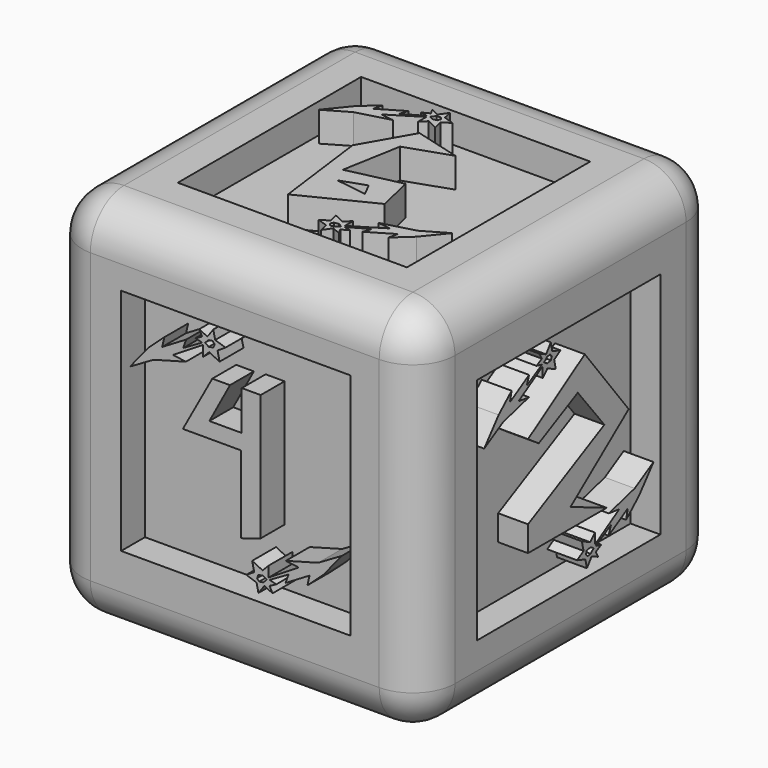
from build123d import *

# Parameters (mm, degrees)
F0_W      = 12.5
F0_H      = 12.5
F1_DEPTH  = 12.5
F2_R      = 1.4103835631
F3_W      = 7.6792328737
F3_H      = 7.6792328737
F4_DEPTH  = 1
F5_W      = 7.6792328737
F5_H      = 7.6792328737
F6_DEPTH  = 1
F7_W      = 7.6792328737
F7_H      = 7.6792328737
F8_DEPTH  = 1
F9_W      = 7.6792328737
F9_H      = 7.6792328737
F10_DEPTH = 1
F12_W     = 7.6792328737
F12_H     = 7.6792328737
F13_DEPTH = 1
F14_W     = 7.6792328737
F14_H     = 7.6792328737
F15_DEPTH = 1


# Not quite as in the source:
# - a feature names something its author has since deleted; it is built from what else it names


with BuildPart() as f1:
    # F0 (on Front) → F1 (new body)
    with BuildSketch(Plane.XZ):
        with Locations((0.0040858053, -0.2807128243)):
            Rectangle(F0_W, F0_H)
    extrude(amount=F1_DEPTH)

    # F2
    f2_edges = [f1.edges().sort_by_distance(p)[0] for p in [
        (-6.245914, -6.25, 5.969287),
        (6.254086, -6.25, 5.969287),
        (0.004086, 0, 5.969287),
        (0.004086, -12.5, 5.969287),
        (-6.245914, -6.25, -6.530713),
        (6.254086, -6.25, -6.530713),
        (0.004086, 0, -6.530713),
        (0.004086, -12.5, -6.530713),
        (6.254086, -12.5, -0.280713),
        (-6.245914, -12.5, -0.280713),
        (6.254086, 0, -0.280713),
        (-6.245914, 0, -0.280713),
    ]]
    fillet(f2_edges, radius=F2_R)

    # F3 (on face) → F4 (cut)
    with BuildSketch(Plane.XY.offset(5.9692871757)):
        with Locations((0.0040858053, -6.25)):
            Rectangle(F3_W, F3_H)
        Polygon((-0.652328541, -3.9411829785), (0.8822005475, -4.3596909381), (-0.5726128584, -4.8579145223), (-0.9213888927, -6.8151349505), (0.8622713503, -6.4123724587), (1.141276909, -7.647966966), (-1.1704812059, -8.8038453832), (-1.5889889328, -5.5753565393), align=None, mode=Mode.SUBTRACT)
        Polygon((3.5567511804, -7.8321555629), (2.9507998843, -8.5790259764), (2.4082618766, -9.0722423047), (2.4787215516, -8.7622206192), (1.6754835378, -9.2413448729), (1.7741267802, -8.959507104), (1.1399915675, -9.325896157), (1.3654618524, -9.3822639901), (1.1399915675, -9.5020448789), (1.2393376978, -9.6890496718), (0.9638429037, -9.5584124792), (0.766556419, -9.83320456), (0.7031428395, -9.5443206374), (0.3578914911, -9.4315854367), (0.6256374181, -9.2624826357), (0.5551779759, -8.9524611831), (0.9074754198, -9.1215639841), (1.1047618464, -8.9172313455), (1.1047618464, -9.2695287894), (2.1193781868, -8.6424394976), (1.6825294588, -8.5860718973), (2.7676052414, -8.2901422866), align=None, mode=Mode.SUBTRACT)
        Polygon((-3.5365826916, -4.553236533), (-2.9306313954, -3.8063661195), (-2.3880933877, -3.3131497912), (-2.4585530628, -3.6231714766), (-1.655315049, -3.144047223), (-1.7539582914, -3.4258849919), (-1.1198230786, -3.0594959389), (-1.3452933636, -3.0031281058), (-1.1198230786, -2.883347217), (-1.2191692089, -2.696342424), (-0.9436744149, -2.8269796167), (-0.7463879301, -2.5521875359), (-0.6829743506, -2.8410714585), (-0.3377230023, -2.9538066592), (-0.6054689293, -3.1229094602), (-0.5350094871, -3.4329309128), (-0.887306931, -3.2638281118), (-1.0845933575, -3.4681607503), (-1.0845933575, -3.1158633064), (-2.0992096979, -3.7429525983), (-1.6623609699, -3.7993201986), (-2.7474367525, -4.0952498093), align=None, mode=Mode.SUBTRACT)
        Polygon((0.7911975845, -9.4897663221), (0.9244724642, -9.4698371831), (1.0452916613, -9.3527548015), (0.918244652, -9.2730389442), (0.7637953386, -9.3004412483), (0.7214463549, -9.4112961087), align=None)
        Polygon((-0.7710290956, -2.8956257738), (-0.9043039754, -2.9155549128), (-1.0251231724, -3.0326372944), (-0.8980761631, -3.1123531517), (-0.7436268497, -3.0849508476), (-0.701277866, -2.9740959872), align=None)
        Polygon((0.3839768178, -7.5283930637), (0.1647583413, -7.0899561979), (-0.6642947193, -7.3738783735), align=None)
    extrude(amount=-F4_DEPTH, mode=Mode.SUBTRACT)

    # F5 (on face) → F6 (cut)
    with BuildSketch(Plane(origin=(0, 0, 0), x_dir=(-1, 0, 0), z_dir=(0, 1, 0))):
        with Locations((-0.1059367728, -0.2820717577)):
            Rectangle(F5_W, F5_H)
        Polygon((3.4467286024, -1.8642273206), (2.8407773062, -2.6110977341), (2.2982392985, -3.1043140624), (2.3686989736, -2.794292377), (1.5654609598, -3.2734166306), (1.6641042022, -2.9915788617), (1.0299689894, -3.3579679147), (1.2554392744, -3.4143357478), (1.0299689894, -3.5341166366), (1.1293151197, -3.7211214296), (0.8538203257, -3.5904842369), (0.6565338409, -3.8652763177), (0.5931202614, -3.5763923951), (0.2478689131, -3.4636571944), (0.5156148401, -3.2945543934), (0.4451553979, -2.9845329408), (0.7974528418, -3.1536357418), (0.9947392683, -2.9493031033), (0.9947392683, -3.3016005472), (2.0093556087, -2.6745112553), (1.5725068807, -2.618143655), (2.6575826633, -2.3222140443), align=None, mode=Mode.SUBTRACT)
        Polygon((-0.8451312315, 1.7336877688), (-0.8451312315, 2.2153509256), (2.2446786681, 0.9617710281), (0.5813771522, -0.5256042938), (1.8385423364, -1.4611691033), (-0.8458287511, -3.1528016366), (-1.0901629205, -2.8107338108), (0.9133041001, -1.3796858916), (-0.5255040818, -0.3914135535), (1.2028907008, 0.4810142225), align=None, mode=Mode.SUBTRACT)
        Polygon((-3.6466052696, 1.4146917093), (-3.0406539735, 2.1615621228), (-2.4981159657, 2.6547784511), (-2.5685756408, 2.3447567656), (-1.765337627, 2.8238810193), (-1.8639808694, 2.5420432504), (-1.2298456567, 2.9084323033), (-1.4553159416, 2.9648001365), (-1.2298456567, 3.0845810253), (-1.329191787, 3.2715858182), (-1.0536969929, 3.1409486256), (-0.8564105082, 3.4157407064), (-0.7929969287, 3.1268567838), (-0.4477455803, 3.0141215831), (-0.7154915073, 2.8450187821), (-0.6450320651, 2.5349973295), (-0.997329509, 2.7041001305), (-1.1946159356, 2.4997674919), (-1.1946159356, 2.8520649358), (-2.209232276, 2.224975644), (-1.772383548, 2.1686080437), (-2.8574593306, 1.872678433), align=None, mode=Mode.SUBTRACT)
        Polygon((-0.8810516737, 3.0723024685), (-1.0143265534, 3.0523733295), (-1.1351457505, 2.9352909479), (-1.0080987412, 2.8555750906), (-0.8536494278, 2.8829773947), (-0.8113004441, 2.9938322551), align=None)
        Polygon((0.6811750064, -3.5218380798), (0.8144498862, -3.5019089408), (0.9352690832, -3.3848265592), (0.8082220739, -3.3051107019), (0.6537727605, -3.3325130061), (0.6114237768, -3.4433678664), align=None)
    extrude(amount=-F6_DEPTH, mode=Mode.SUBTRACT)

    # F7 (on face) → F8 (cut)
    with BuildSketch(Plane(origin=(0, 0, -6.5307128243), x_dir=(1, 0, 0), z_dir=(0, 0, -1))):
        with Locations((0.0040858053, 6.25)):
            Rectangle(F7_W, F7_H)
        Polygon((3.7880760211, 4.7270533688), (3.182124725, 3.9801829554), (2.6395867172, 3.4869666271), (2.7100463923, 3.7969883125), (1.9068083785, 3.3178640589), (2.0054516209, 3.5997018277), (1.3713164082, 3.2333127748), (1.5967866931, 3.1769449416), (1.3713164082, 3.0571640529), (1.4706625385, 2.8701592599), (1.1951677444, 3.0007964525), (0.9978812597, 2.7260043718), (0.9344676802, 3.0148882944), (0.5892163318, 3.1276234951), (0.8569622588, 3.2967262961), (0.7865028166, 3.6067477487), (1.1388002605, 3.4376449477), (1.3360866871, 3.6419775862), (1.3360866871, 3.2896801423), (2.3507030274, 3.9167694341), (1.9138542995, 3.9731370345), (2.9989300821, 4.2690666452), align=None, mode=Mode.SUBTRACT)
        Polygon((-0.234052015, 8.3048082888), (-0.8038301021, 8.3048082888), (0, 9.1091999784), (0.5368242273, 9.1091999784), (0.5368242273, 3.8303739857), (-0.234052015, 3.8303739857), align=None, mode=Mode.SUBTRACT)
        Polygon((-3.7074539285, 7.7881164908), (-3.1015026324, 8.5349869042), (-2.5589646247, 9.0282032326), (-2.6294242997, 8.7181815471), (-1.8261862859, 9.1973058007), (-1.9248295283, 8.9154680319), (-1.2906943156, 9.2818570848), (-1.5161646005, 9.338224918), (-1.2906943156, 9.4580058068), (-1.3900404459, 9.6450105997), (-1.1145456518, 9.5143734071), (-0.9172591671, 9.7891654879), (-0.8538455876, 9.5002815652), (-0.5085942392, 9.3875463646), (-0.7763401662, 9.2184435636), (-0.705880724, 8.908422111), (-1.0581781679, 9.077524912), (-1.2554645945, 8.8731922734), (-1.2554645945, 9.2254897173), (-2.2700809349, 8.5984004255), (-1.8332322069, 8.5420328252), (-2.9183079895, 8.2461032145), align=None, mode=Mode.SUBTRACT)
        Polygon((-0.9419003326, 9.44572725), (-1.0751752123, 9.425798111), (-1.1959944094, 9.3087157294), (-1.0689474001, 9.2289998721), (-0.9144980867, 9.2564021762), (-0.872149103, 9.3672570366), align=None)
        Polygon((1.0225224252, 3.0694426097), (1.1557973049, 3.0893717486), (1.276616502, 3.2064541302), (1.1495694927, 3.2861699875), (0.9951201793, 3.2587676834), (0.9527711956, 3.147912823), align=None)
    extrude(amount=-F8_DEPTH, mode=Mode.SUBTRACT)

    # F9 (on face) → F10 (cut)
    with BuildSketch(Plane.XZ.offset(12.5)):
        with Locations((0.0344234001, -0.0645021169)):
            Rectangle(F9_W, F9_H)
        Polygon((3.5870887752, -1.6466576798), (2.9811374791, -2.3935280932), (2.4385994714, -2.8867444215), (2.5090591464, -2.5767227361), (1.7058211326, -3.0558469897), (1.804464375, -2.7740092209), (1.1703291623, -3.1403982738), (1.3957994472, -3.196766107), (1.1703291623, -3.3165469958), (1.2696752926, -3.5035517887), (0.9941804985, -3.3729145961), (0.7968940138, -3.6477066768), (0.7334804343, -3.3588227542), (0.3882290859, -3.2460875535), (0.6559750129, -3.0769847525), (0.5855155707, -2.7669632999), (0.9378130146, -2.9360661009), (1.1350994412, -2.7317334624), (1.1350994412, -3.0840309063), (2.1497157816, -2.4569416145), (1.7128670536, -2.4005740141), (2.7979428362, -2.1046444034), align=None, mode=Mode.SUBTRACT)
        Polygon((-1.7355565215, 0.3694626794), (-0.7491240976, 2.1732251626), (-0.1572645706, 2.1732251626), (-0.84776734, 0.8908626623), (0.2373084135, 0.8908626623), (0.2373084135, 2.2155006882), (0.8714435971, 2.2155006882), (0.8714435971, -2.0120672416), (0.209124657, -2.2234455682), (0.209124657, 0.3694626794), align=None, mode=Mode.SUBTRACT)
        Polygon((-3.5062450968, 1.6322613502), (-2.9002938006, 2.3791317636), (-2.3577557929, 2.8723480919), (-2.428215468, 2.5623264065), (-1.6249774542, 3.0414506601), (-1.7236206966, 2.7596128913), (-1.0894854838, 3.1260019442), (-1.3149557688, 3.1823697774), (-1.0894854838, 3.3021506662), (-1.1888316141, 3.4891554591), (-0.9133368201, 3.3585182665), (-0.7160503353, 3.6333103472), (-0.6526367558, 3.3444264246), (-0.3073854075, 3.2316912239), (-0.5751313345, 3.0625884229), (-0.5046718923, 2.7525669703), (-0.8569693362, 2.9216697713), (-1.0542557627, 2.7173371328), (-1.0542557627, 3.0696345767), (-2.0688721031, 2.4425452849), (-1.6320233751, 2.3861776846), (-2.7170991577, 2.0902480738), align=None, mode=Mode.SUBTRACT)
        Polygon((-0.7406915008, 3.2898721093), (-0.8739663806, 3.2699429704), (-0.9947855776, 3.1528605888), (-0.8677385683, 3.0731447315), (-0.7132892549, 3.1005470356), (-0.6709402712, 3.211401896), align=None)
        Polygon((0.8215351793, -3.3042684389), (0.954810059, -3.2843393), (1.0756292561, -3.1672569184), (0.9485822468, -3.0875410611), (0.7941329334, -3.1149433652), (0.7517839497, -3.2257982256), align=None)
    extrude(amount=-F10_DEPTH, mode=Mode.SUBTRACT)


with BuildPart() as f1_1:
    # F11: moved
    add(f1.part.moved(Location((0, 6.25005, 0.28075))))

    # F12 (on face) → F13 (cut)
    with BuildSketch(Plane.YZ.offset(6.2540858053)):
        with Locations((-0.0755139039, -0.0997889451)):
            Rectangle(F12_W, F12_H)
        Polygon((3.4771514713, -1.6819445081), (2.8712001751, -2.4288149215), (2.3286621674, -2.9220312498), (2.3991218425, -2.6120095644), (1.5958838287, -3.091133818), (1.6945270711, -2.8092960491), (1.0603918583, -3.1756851021), (1.2858621433, -3.2320529352), (1.0603918583, -3.351833824), (1.1597379886, -3.538838617), (0.8842431946, -3.4082014244), (0.6869567098, -3.6829935051), (0.6235431304, -3.3941095825), (0.278291782, -3.2813743818), (0.546037709, -3.1122715808), (0.4755782668, -2.8022501282), (0.8278757107, -2.9713529292), (1.0251621372, -2.7670202907), (1.0251621372, -3.1193177346), (2.0397784776, -2.4922284428), (1.6029297496, -2.4358608424), (2.6880055323, -2.1399312317), align=None, mode=Mode.SUBTRACT)
        Polygon((-3.6161824007, 1.5969745219), (-3.0102311046, 2.3438449353), (-2.4676930968, 2.8370612637), (-2.5381527719, 2.5270395782), (-1.7349147581, 3.0061638318), (-1.8335580005, 2.724326063), (-1.1994227878, 3.0907151159), (-1.4248930727, 3.1470829491), (-1.1994227878, 3.2668638379), (-1.2987689181, 3.4538686308), (-1.023274124, 3.3232314382), (-0.8259876393, 3.598023519), (-0.7625740598, 3.3091395963), (-0.4173227114, 3.1964043957), (-0.6850686384, 3.0273015947), (-0.6146091962, 2.717280142), (-0.9669066401, 2.8863829431), (-1.1641930667, 2.6820503045), (-1.1641930667, 3.0343477484), (-2.1788094071, 2.4072584566), (-1.7419606791, 2.3508908563), (-2.8270364617, 2.0549612455), align=None, mode=Mode.SUBTRACT)
        Polygon((-1.3304492459, 0.8229081286), (-1.7807424301, 1.1310036061), (0.5976638724, 2.6675111191), (2.4377943482, 0.3015158582), (0, -1.5944556799), (1.5135082649, -2.2343462333), (-1.7807424301, -2.2343462333), (-1.7807424301, -1.3811589452), (1.4187095221, 0.2541166323), (0.3048262151, 1.652395702), align=None, mode=Mode.SUBTRACT)
        Polygon((-0.8506288048, 3.2545852811), (-0.9839036845, 3.2346561421), (-1.1047228816, 3.1175737605), (-0.9776758723, 3.0378579032), (-0.8232265589, 3.0652602073), (-0.7808775752, 3.1761150677), align=None)
        Polygon((0.7115978753, -3.3395552672), (0.8448727551, -3.3196261283), (0.9656919522, -3.2025437466), (0.8386449429, -3.1228278894), (0.6841956294, -3.1502301935), (0.6418466457, -3.2610850539), align=None)
    extrude(amount=-F13_DEPTH, mode=Mode.SUBTRACT)

    # F14 (on face) → F15 (cut)
    with BuildSketch(Plane(origin=(-6.2459141947, 0, 0), x_dir=(0, -1, 0), z_dir=(-1, 0, 0))):
        with Locations((0.040559386, 0.0628033146)):
            Rectangle(F14_W, F14_H)
        Polygon((-1.527969609, 0), (-1.527969609, 1.9783561584), (1.2022961164, 2.0780009218), (0.6442855811, 1.4602035517), (-0.9699591319, 1.4602035517), (-0.6956497673, 0), (0.4449960252, -0.4330463416), (1.0827222141, -1.6088541597), (0.1659907575, -2.3462250829), (-1.527969609, -2.3462250829), (-1.527969609, -1.5689962311), (0, -1.3697067043), align=None, mode=Mode.SUBTRACT)
        Polygon((3.5932247612, -1.5193522483), (2.987273465, -2.2662226618), (2.4447354573, -2.7594389901), (2.5151951323, -2.4494173046), (1.7119571186, -2.9285415583), (1.8106003609, -2.6467037894), (1.1764651482, -3.0130928423), (1.4019354331, -3.0694606755), (1.1764651482, -3.1892415643), (1.2758112785, -3.3762463572), (1.0003164844, -3.2456091646), (0.8030299997, -3.5204012454), (0.7396164202, -3.2315173228), (0.3943650719, -3.1187821221), (0.6621109988, -2.9496793211), (0.5916515566, -2.6396578685), (0.9439490005, -2.8087606695), (1.1412354271, -2.6044280309), (1.1412354271, -2.9567254748), (2.1558517675, -2.329636183), (1.7190030395, -2.2732685827), (2.8040788221, -1.977338972), align=None, mode=Mode.SUBTRACT)
        Polygon((-3.5001091109, 1.7595667816), (-2.8941578147, 2.5064371951), (-2.351619807, 2.9996535234), (-2.422079482, 2.689631838), (-1.6188414683, 3.1687560916), (-1.7174847107, 2.8869183227), (-1.0833494979, 3.2533073757), (-1.3088197828, 3.3096752088), (-1.0833494979, 3.4294560976), (-1.1826956282, 3.6164608906), (-0.9072008342, 3.4858236979), (-0.7099143494, 3.7606157787), (-0.6465007699, 3.4717318561), (-0.3012494216, 3.3589966554), (-0.5689953486, 3.1898938544), (-0.4985359063, 2.8798724018), (-0.8508333502, 3.0489752028), (-1.0481197768, 2.8446425643), (-1.0481197768, 3.1969400082), (-2.0627361172, 2.5698507163), (-1.6258873892, 2.513483116), (-2.7109631718, 2.2175535053), align=None, mode=Mode.SUBTRACT)
        Polygon((-0.7345555149, 3.4171775408), (-0.8678303947, 3.3972484018), (-0.9886495917, 3.2801660202), (-0.8616025824, 3.2004501629), (-0.707153269, 3.2278524671), (-0.6648042853, 3.3387073274), align=None)
        Polygon((0.8276711652, -3.1769630075), (0.960946045, -3.1570338685), (1.081765242, -3.0399514869), (0.9547182327, -2.9602356296), (0.8002689193, -2.9876379337), (0.7579199356, -3.0984927941), align=None)
    extrude(amount=-F15_DEPTH, mode=Mode.SUBTRACT)


solid = f1_1.part
